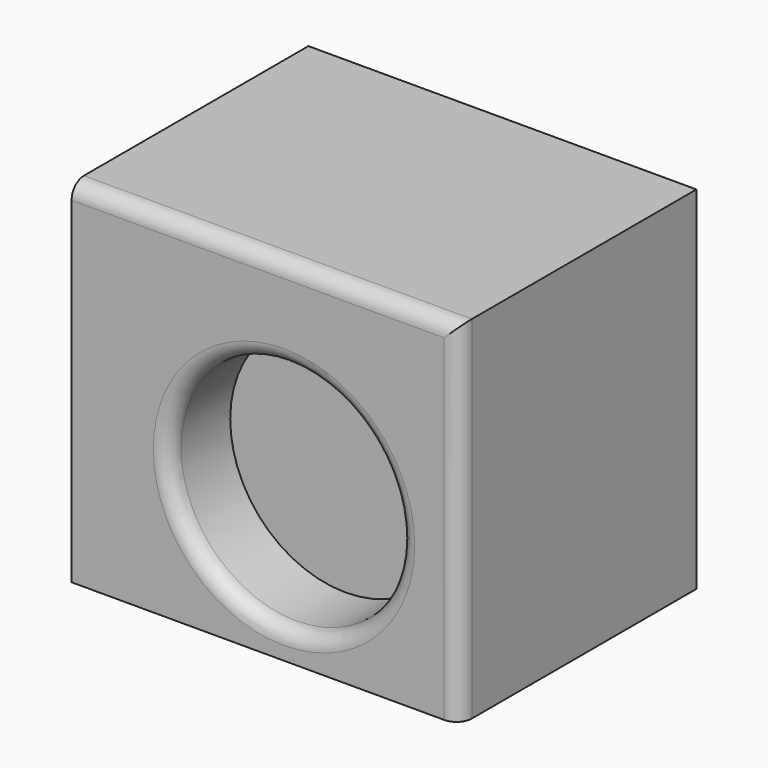
from build123d import *

# Parameters (mm, degrees)
F0_W     = 128.2316669822
F0_H     = 97.8200212121
F1_DEPTH = 116.2282433361
F2_R     = 38.1
F3_DEPTH = 25.4
F4_R     = 5.08


with BuildPart() as f1:
    # F0 (on Top) → F1 (new body)
    with BuildSketch(Plane.XY):
        with Locations((7.463093847, 4.6752728522)):
            Rectangle(F0_W, F0_H)
    extrude(amount=F1_DEPTH)

    # F2 (on face) → F3 (cut)
    with BuildSketch(Plane.XZ.offset(44.2347377539)):
        with Locations((13.5555826128, 47.6286895573)):
            Circle(F2_R)
    extrude(amount=-F3_DEPTH, mode=Mode.SUBTRACT)

    # F4
    f4_edges = [f1.edges().sort_by_distance(p)[0] for p in [
        (71.578927, -44.234738, 58.114122),
        (7.463094, -44.234738, 116.228243),
        (-24.544417, -44.234738, 47.62869),
    ]]
    fillet(f4_edges, radius=F4_R)


solid = f1.part
